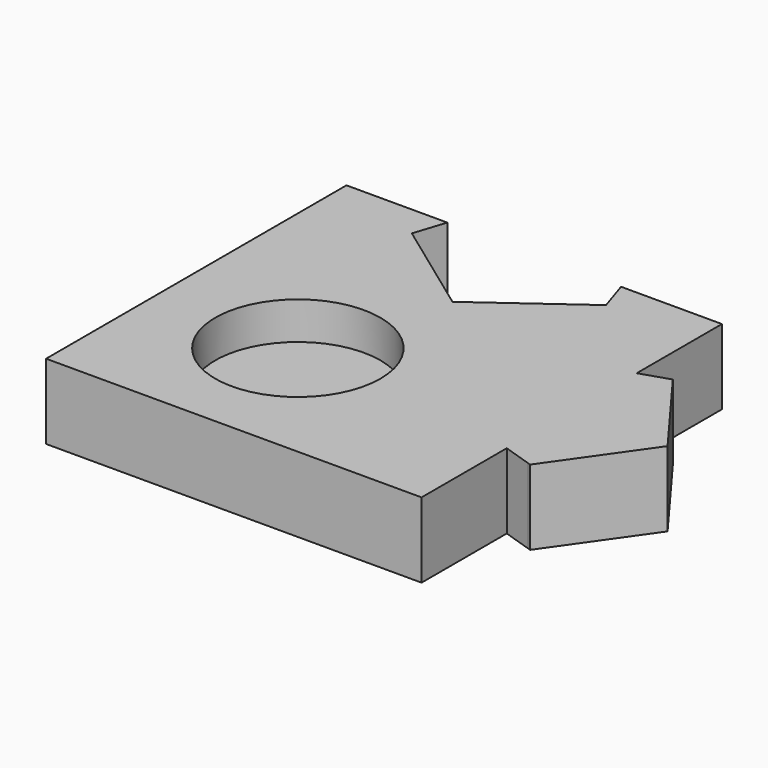
from build123d import *

# Parameters (mm, degrees)
F1_DEPTH = 10
F2_R     = 11
F3_DEPTH = 5


# Not quite as in the source:
# - a feature names something its author has since deleted; it is built from what else it names


with BuildPart() as f1:
    # F0 (on Top) → F1 (new body)
    with BuildSketch(Plane.XY):
        Polygon((-25, -25), (25, -25), (25, -10.8146222424), (25, -10.5146222424), (15, -7.2654252801), (15, 7.2654252801), (25, 10.5146222424), (25, 10.8146222424), (25, 25), (11.5660844666, 25), (12.9312755504, 20.7983738762), (0, 11.4032522475), (-12.9312755504, 20.7983738762), (-11.5660844666, 25), (-25, 25), align=None)
        Polygon((25, 10.5146222424), (25, -10.5146222424), (28.8196601125, -11.7557050458), (37.360679775, 0), (28.8196601125, 11.7557050458), align=None)
        Polygon((15, -7.2654252801), (25, -10.5146222424), (25, 10.5146222424), (15, 7.2654252801), align=None)
        Polygon((25, 10.8146222424), (25, 10.5146222424), (28.8196601125, 11.7557050458), (37.360679775, 0), (37.760679775, 0), (28.8196601125, 12.0557050458), align=None)
        Polygon((25, -10.5146222424), (25, -10.8146222424), (28.8196601125, -12.0557050458), (29.200082719, -12.1793118436), (37.760679775, 0), (37.360679775, 0), (28.8196601125, -11.7557050458), align=None)
    extrude(amount=F1_DEPTH)

    # F2 (on face) → F3 (cut)
    with BuildSketch(Plane.XY.offset(10)):
        with Locations((-6.0343622248, -6.7983738762)):
            Circle(F2_R)
    extrude(amount=-F3_DEPTH, mode=Mode.SUBTRACT)


solid = f1.part
